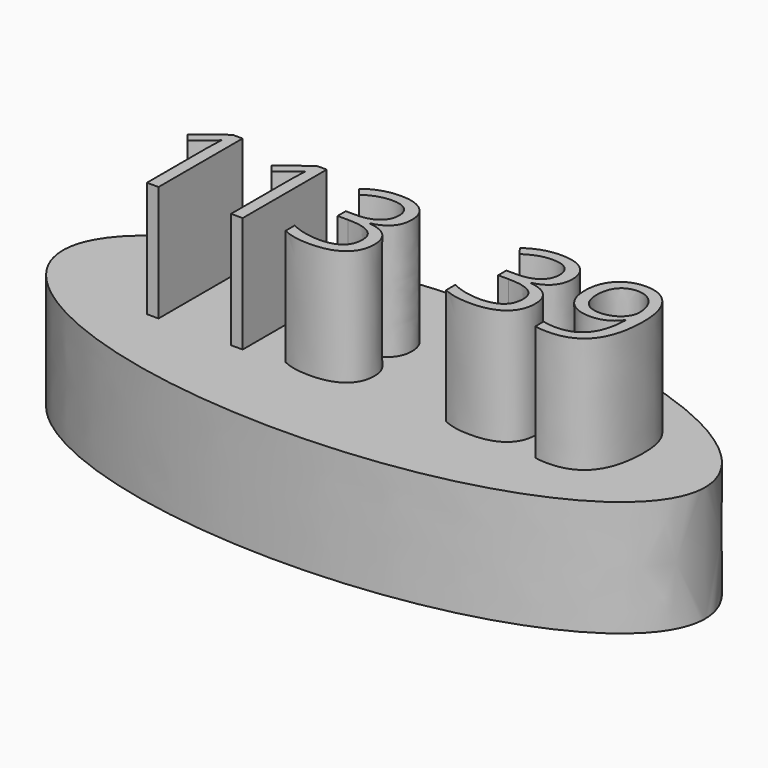
from build123d import *

# Parameters (mm, degrees)
F1_DEPTH     = 25.4
F2_TEXT_SIZE = 32.2974144688
F3_DEPTH     = 25.4


# Not quite as in the source:
# - Text() gives the source's letters only with a copy of the font that has no kerning and outlines rounded to 1/6400 em; it was checked with that copy


with BuildPart() as f1:
    # F0 (on Top) → F1 (new body)
    with BuildSketch(Plane.XY):
        with BuildLine():
            add(Edge.make_bspline(
                [(70.4521536827, 0), (70.4521536827, 50.1394808772), (-35.2260768414, 25.0697404386), (-140.9043073654, 0), (-35.2260768414, -25.0697404386), (70.4521536827, -50.1394808772), (70.4521536827, 0)],
                knots=[0, 0, 0, 2.0943951024, 2.0943951024, 4.1887902048, 4.1887902048, 6.2831853072, 6.2831853072, 6.2831853072], degree=2, weights=[1, 0.5, 1, 0.5, 1, 0.5, 1]))
        make_face()
    extrude(amount=F1_DEPTH)

    # F2 (on face) → F3 (join)
    with BuildSketch(Plane.XY.offset(25.4)):
        with Locations((-53.1100863591, -9.5578460023)):
            Text('113  39', F2_TEXT_SIZE, font='Open Sans', text_align=(TextAlign.LEFT, TextAlign.BOTTOM))
    extrude(amount=F3_DEPTH)


solid = f1.part
